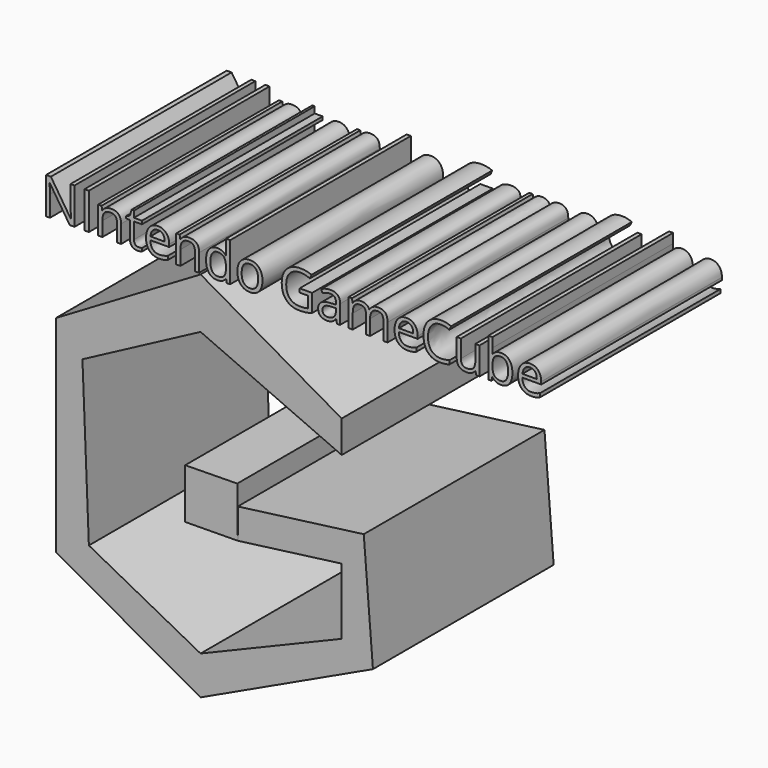
from build123d import *

# Parameters (mm, degrees)
F1_DEPTH     = 76.2
F3_DEPTH     = 76.2
F4_TEXT_SIZE = 17.2286708322
F5_DEPTH     = 76.2


# Not quite as in the source:
# - Text() gives the source's letters only with a copy of the font that has no kerning and outlines rounded to 1/6400 em; it was checked with that copy


with BuildPart() as f1:
    # F0 (on Front) → F1 (new body)
    with BuildSketch(Plane.XZ):
        Polygon((47.6028472185, 26.8250592053), (0, 54.1152916849), (-48.8433167338, 25.2744778991), (-48.8433167338, -44.1915728152), (0, -71.4818015695), (58.1467971206, -44.1915728152), (55.0456382334, -5.1169185899), (12.5597100705, -10.6990123168), (12.5597100705, -20.8853123204), (47.6028472185, -16.2811037153), (47.6028472185, -38.6094748974), (0, -58.4569200873), (-37.6791283488, -38.6094748974), (-39.8499406874, 15.9709881991), (0, 37.0588973165), (47.6028472185, 15.9709881991), align=None)
    extrude(amount=F1_DEPTH)


with BuildPart() as f3:
    # F2 (on face) → F3 (new body)
    with BuildSketch(Plane.XZ.offset(76.2)):
        Polygon((12.3753304057, -3.9614559419), (-5.1879156381, -4.2106839828), (-5.1879156381, -21.0786666721), (12.5597100705, -20.8853123204), align=None)
    extrude(amount=-F3_DEPTH)


with BuildPart() as f5:
    # F4 (on Front) → F5 (new body)
    with BuildSketch(Plane.XZ):
        with Locations((-53.8051761687, 54.4254109263)):
            Text('NIntendo GameCube', F4_TEXT_SIZE, font='Open Sans', text_align=(TextAlign.LEFT, TextAlign.BOTTOM))
    extrude(amount=F5_DEPTH)


solid = Compound([f1.part, f3.part, f5.part])
